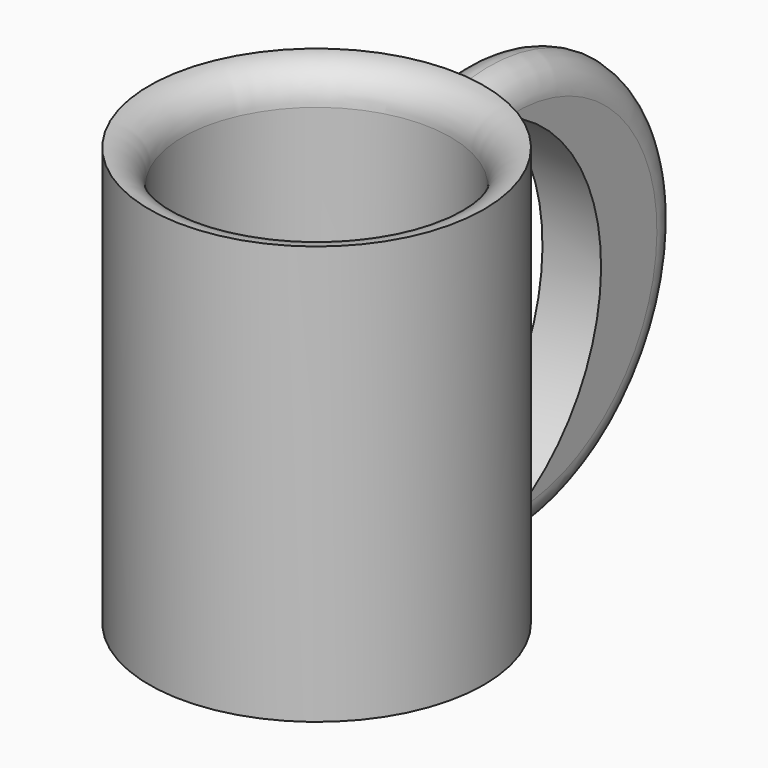
from build123d import *

# Parameters (mm, degrees)
F0_R         = 50.8
F1_DEPTH     = 127
F2_T         = -10.16
F5_DEPTH     = 8.89
F6_T4_ANGLE  = 254.7462790776
F6_S5_R      = 50.8
F6_T6_DEPTH  = 89
F6_T11_ANGLE = 254.7462790776
F6_S12_R     = 50.8
F6_T13_DEPTH = 89
F6_T18_ANGLE = 254.7462790776
F6_S19_R     = 50.8
F6_T20_DEPTH = 89
F7_T4_ANGLE  = 254.3575983754
F7_S5_R      = 50.8
F7_T6_DEPTH  = 89
F7_T10_ANGLE = 254.3575983754


# Not quite as in the source:
# - a fillet or chamfer that OpenCascade refuses, or shapes differently, is made with other operations: its cross-section is extruded or revolved along the edge and cut away or added


with BuildPart() as f1:
    # F0 (on Top) → F1 (new body)
    with BuildSketch(Plane.XY):
        Circle(F0_R)
    extrude(amount=F1_DEPTH)

    # F2
    f2_openings = [f1.faces().sort_by_distance(p)[0] for p in [
        (0, 0, 127),
    ]]
    offset(amount=F2_T, openings=f2_openings)

    # F3: fillet of radius 10.4245741623 on 1 edges, made by hand

    # F3_s1 → F3_t2 (revolve, cut)
    with BuildSketch(Plane.XZ):
        with BuildLine():
            ThreePointArc((50.8, 127), (43.6003320895, 123.8559286261), (40.64, 116.5787838052))
            Line((40.64, 116.5787838052), (40.64, 127))
            Line((40.64, 127), (50.8, 127))
        make_face()
    revolve(axis=Axis((0, 0, 127), (0, 0, 1)), mode=Mode.SUBTRACT)

    # F4 (on Right) → F5 (join, symmetric)
    with BuildSketch(Plane.YZ):
        with BuildLine():
            ThreePointArc((40.9011468769, 118.0027031276), (96.7316605485, 61.0144931984), (45.3319139779, 0))
            ThreePointArc((45.3319139779, 0), (127.3418829144, 62.1638462438), (40.9011468769, 118.0027031276))
        make_face()
    extrude(amount=F5_DEPTH, both=True)

    # F6: fillet of radius 9.525 on 1 edges, made by hand


with BuildPart() as f6_tool2:
    # F6_s3 → F6_t4 (revolve)
    with BuildSketch(Plane(origin=(0, 8.968139316, -7.4168504874), x_dir=(1, 0, 0), z_dir=(0, -0.7706077503, 0.6373097325))):
        with BuildLine():
            ThreePointArc((-8.89, 33.9367221949), (-6.1001920908, 27.2015301041), (0.635, 24.4117221949))
            Line((0.635, 24.4117221949), (-8.89, 24.4117221949))
            Line((-8.89, 24.4117221949), (-8.89, 33.9367221949))
        make_face()
    revolve(axis=Axis((-8.89, 64.5634606481, 59.8066411912), (1, 0, 0)), revolution_arc=F6_T4_ANGLE)

    # F6_s5 → F6_t6 (intersect, symmetric)
    with BuildSketch(Plane.XY.offset(59.8)):
        Circle(F6_S5_R)
    extrude(amount=F6_T6_DEPTH, both=True, mode=Mode.INTERSECT)

    split(bisect_by=Plane.XY, keep=Keep.BOTTOM)


with BuildPart() as f1_1:
    add(f1.part)

    # F6_t1: cut F6_tool2
    add(f6_tool2.part, mode=Mode.SUBTRACT)


with BuildPart() as f6_tool9:
    # F6_s10 → F6_t11 (revolve)
    with BuildSketch(Plane(origin=(0, 8.968139316, -7.4168504874), x_dir=(1, 0, 0), z_dir=(0, -0.7706077503, 0.6373097325))):
        with BuildLine():
            ThreePointArc((-8.89, 33.9367221949), (-6.1001920908, 27.2015301041), (0.635, 24.4117221949))
            Line((0.635, 24.4117221949), (-8.89, 24.4117221949))
            Line((-8.89, 24.4117221949), (-8.89, 33.9367221949))
        make_face()
    revolve(axis=Axis((-8.89, 64.5634606481, 59.8066411912), (1, 0, 0)), revolution_arc=F6_T11_ANGLE)

    # F6_s12 → F6_t13 (cut, symmetric)
    with BuildSketch(Plane.XY.offset(59.8)):
        Circle(F6_S12_R)
    extrude(amount=F6_T13_DEPTH, both=True, mode=Mode.SUBTRACT)

    split(bisect_by=Plane.XY, keep=Keep.TOP)


with BuildPart() as f1_2:
    add(f1_1.part)

    # F6_t8: cut F6_tool9
    add(f6_tool9.part, mode=Mode.SUBTRACT)


with BuildPart() as f6_tool16:
    # F6_s17 → F6_t18 (revolve)
    with BuildSketch(Plane(origin=(0, 8.968139316, -7.4168504874), x_dir=(1, 0, 0), z_dir=(0, -0.7706077503, 0.6373097325))):
        with BuildLine():
            ThreePointArc((-8.89, 33.9367221949), (-6.1001920908, 27.2015301041), (0.635, 24.4117221949))
            Line((0.635, 24.4117221949), (-8.89, 24.4117221949))
            Line((-8.89, 24.4117221949), (-8.89, 33.9367221949))
        make_face()
    revolve(axis=Axis((-8.89, 64.5634606481, 59.8066411912), (1, 0, 0)), revolution_arc=F6_T18_ANGLE)

    # F6_s19 → F6_t20 (cut, symmetric)
    with BuildSketch(Plane.XY.offset(59.8)):
        Circle(F6_S19_R)
    extrude(amount=F6_T20_DEPTH, both=True, mode=Mode.SUBTRACT)

    split(bisect_by=Plane.XY, keep=Keep.BOTTOM)


with BuildPart() as f1_3:
    add(f1_2.part)

    # F6_t15: cut F6_tool16
    add(f6_tool16.part, mode=Mode.SUBTRACT)

    # F7: fillet of radius 9.525 on 1 edges, made by hand


with BuildPart() as f7_tool2:
    # F7_s3 → F7_t4 (revolve)
    with BuildSketch(Plane(origin=(0, 9.2218448194, -7.5741443116), x_dir=(1, 0, 0), z_dir=(0, -0.7727649908, 0.6346922632))):
        with BuildLine():
            ThreePointArc((0.635, 24.3717466269), (6.5351595171, 27.541577675), (8.89, 33.8117002814))
            Line((8.89, 33.8117002814), (8.89, 24.3717466269))
            Line((8.89, 24.3717466269), (0.635, 24.3717466269))
        make_face()
    revolve(axis=Axis((8.89, 64.5634606481, 59.8066411912), (1, 0, 0)), revolution_arc=F7_T4_ANGLE)

    # F7_s5 → F7_t6 (cut, symmetric)
    with BuildSketch(Plane.XY.offset(59.8)):
        Circle(F7_S5_R)
    extrude(amount=F7_T6_DEPTH, both=True, mode=Mode.SUBTRACT)


with BuildPart() as f1_4:
    add(f1_3.part)

    # F7_t1: cut F7_tool2
    add(f7_tool2.part, mode=Mode.SUBTRACT)


with BuildPart() as f7_tool8:
    # F7_s9 → F7_t10 (revolve)
    with BuildSketch(Plane(origin=(0, 9.2218448194, -7.5741443116), x_dir=(1, 0, 0), z_dir=(0, -0.7727649908, 0.6346922632))):
        with BuildLine():
            ThreePointArc((0.635, 24.3717466269), (6.5351595171, 27.541577675), (8.89, 33.8117002814))
            Line((8.89, 33.8117002814), (8.89, 24.3717466269))
            Line((8.89, 24.3717466269), (0.635, 24.3717466269))
        make_face()
    revolve(axis=Axis((8.89, 64.5634606481, 59.8066411912), (1, 0, 0)), revolution_arc=F7_T10_ANGLE)

    split(bisect_by=Plane.XY, keep=Keep.BOTTOM)


with BuildPart() as f1_5:
    add(f1_4.part)

    # F7_t7: cut F7_tool8
    add(f7_tool8.part, mode=Mode.SUBTRACT)


solid = f1_5.part
